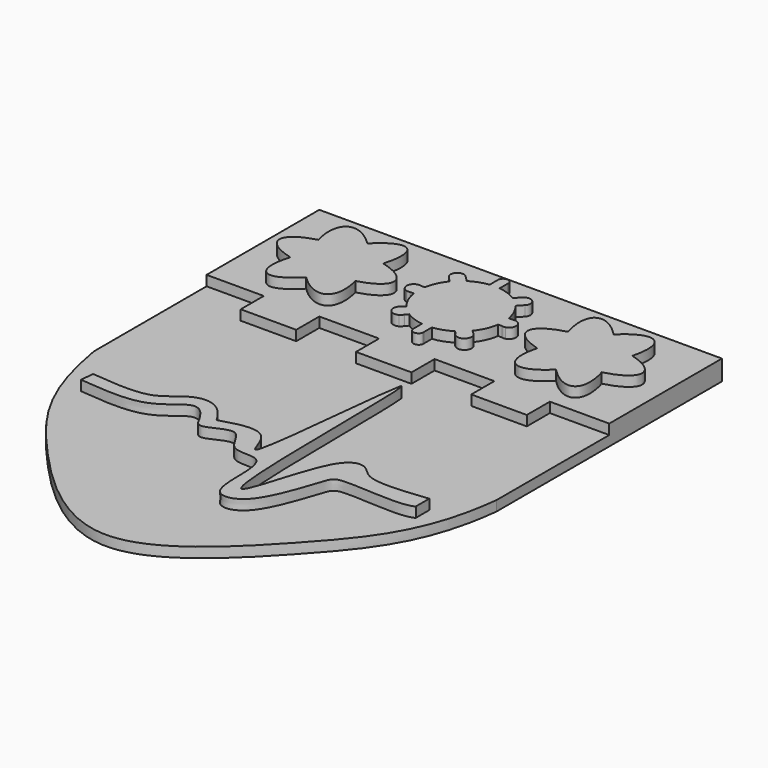
from build123d import *

# Parameters (mm, degrees)
F1_W     = 39.9420261383
F1_H     = 27.9453219846
F2_DEPTH = 1
F4_DEPTH = 1
F6_DEPTH = 1


# Not quite as in the source:
# - the dataset's text gives a spline's control points without its knots; the knots are read off the source's solid


with BuildPart() as f2:
    # F1 (on Top) → F2 (new body)
    with BuildSketch(Plane.XY):
        with Locations((-83.5190042853, -4.0500960313)):
            Rectangle(F1_W, F1_H)
        with BuildLine():
            Line((-63.5479912162, -18.0227570236), (-103.4900173545, -18.0227570236))
            add(Edge.make_bspline(
                [(-103.4900173545, -18.0227570236), (-102.2234410048, -25.4669263959), (-97.486988461, -32.1768391347), (-83.4606816135, -46.0047948801), (-69.8215316304, -32.1663174955), (-64.4036382437, -25.4669263959), (-63.5479912162, -18.0227570236)],
                knots=[0, 0, 0, 0, 0.2558847419, 0.5000748483, 0.7439617176, 1, 1, 1, 1], degree=3))
        make_face()
    extrude(amount=F2_DEPTH)

    # F3 (on face) → F4 (join)
    with BuildSketch(Plane.XY.offset(1)):
        Polygon((-63.5479912162, -4.0500960313), (-63.5479912162, 9.922564961), (-103.4900173545, 9.922564961), (-103.4900173545, -4.0500960313), (-97.8155806661, -4.0500960313), (-97.8155806661, -6.9113592617), (-92.309743166, -6.9113592617), (-92.309743166, -4.0500960313), (-86.3803848624, -4.0500960313), (-86.3803848624, -6.9113592617), (-80.8745473623, -6.9113592617), (-80.8745473623, -4.0500960313), (-74.9451816082, -4.0500960313), (-74.9451816082, -6.9113592617), (-69.4393441081, -6.9113592617), (-69.4393441081, -4.0500960313), align=None)
        with BuildLine():
            add(Edge.make_bspline(
                [(-99.9630689621, -22.528225556), (-97.8050084092, -22.7383123223), (-94.1912663782, -23.0901093914), (-92.2422886498, -20.9561810285), (-90.3592675898, -20.2382765916), (-88.6710398016, -21.005893073), (-88.0005728108, -22.0533678663), (-87.6555964351, -22.5923266262)],
                knots=[0, 0, 0, 0, 0.2982120175, 0.4993656458, 0.66799691, 0.8291739574, 1, 1, 1, 1], degree=3))
            Line((-99.9630689621, -22.528225556), (-100.0935046569, -23.8680916157))
            add(Edge.make_bspline(
                [(-100.0935046569, -23.8680916157), (-99.641213077, -23.9121221112), (-98.7256666906, -24.0013256025), (-97.3584195596, -24.0992161028), (-96.2496019484, -24.1156934281), (-95.3896884341, -24.0638057393), (-94.7581929451, -23.9828672575), (-94.1422492867, -23.8502276061), (-93.5344705995, -23.6422045902), (-93.006004873, -23.3810911586), (-92.5512837964, -23.0968639007), (-92.1638061399, -22.8137321841), (-91.8333347735, -22.5526394177), (-91.5990504655, -22.367477718), (-91.4335751937, -22.2442966641), (-91.3220361628, -22.1663504456), (-91.2159956347, -22.0984600773), (-91.0759198908, -22.0169760478), (-90.9085588347, -21.9349451245), (-90.7257093459, -21.8681143195), (-90.5668189159, -21.8310155496), (-90.4352776818, -21.8190847483), (-90.290771702, -21.8270624276), (-90.0603195544, -21.8881208906), (-89.8056183823, -22.0372246709), (-89.6190164707, -22.1952265623), (-89.420072284, -22.4014685652), (-89.1509209686, -22.7543702908), (-88.9156376248, -23.1208761097), (-88.789421369, -23.3180645593)],
                knots=[0, 0, 0, 0, 0.0625, 0.125, 0.1875, 0.21875, 0.25, 0.28125, 0.3125, 0.34375, 0.375, 0.40625, 0.4375, 0.46875, 0.484375, 0.5, 0.515625, 0.53125, 0.5625, 0.59375, 0.625, 0.65625, 0.6875, 0.75, 0.8125, 0.84375, 0.875, 0.9375, 1, 1, 1, 1], degree=3))
            add(Edge.make_bspline(
                [(-88.789421369, -23.3180645593), (-88.6064399588, -23.7055464069), (-88.1334203276, -24.7072138465), (-84.8867718058, -22.1498784727), (-84.1139103536, -26.1676816962), (-80.4918087102, -24.9787016454), (-80.5104213919, -29.1352666664), (-80.3521996357, -32.500651404), (-76.6927369801, -31.9827435011), (-74.8542261683, -25.2740014974), (-74.103136335, -24.0138444224), (-67.6515141347, -24.9719990423), (-66.5661245584, -24.263119325)],
                knots=[0, 0, 0, 0, 0.0560038879, 0.1447739329, 0.2315937968, 0.3157568277, 0.4138471485, 0.5050737567, 0.5873258169, 0.7241585594, 0.7883299015, 0.9309694647, 0.9309694647, 0.9309694647, 0.9309694647], degree=3))
            Line((-66.5661245584, -24.263119325), (-66.566221416, -22.5923266262))
            add(Edge.make_bspline(
                [(-87.6555964351, -22.5923266262), (-85.892468446, -22.0624948678), (-82.88294857, -21.1581140072), (-81.8661255421, -28.9674864594), (-79.189868147, 7.6035712637), (-80.2972010381, -41.1991140851), (-76.7122142141, -21.5352294093), (-73.6666754342, -21.215900503), (-72.5063764781, -23.2421096322), (-68.8986686121, -22.84746888), (-66.566221416, -22.5923266262)],
                knots=[0, 0, 0, 0, 0.1037610874, 0.1771119606, 0.3711377094, 0.59782823, 0.7400426838, 0.8156894581, 0.880839962, 1, 1, 1, 1], degree=3))
        make_face()
    extrude(amount=F4_DEPTH)

    # F5 (on face) → F6 (join)
    with BuildSketch(Plane.XY.offset(2)):
        with BuildLine():
            Line((-84.1366667768, 7.8781278824), (-84.1366667768, 6.858777233))
            ThreePointArc((-84.1366667768, 6.858777233), (-85.0572011542, 6.6404288094), (-85.9061185607, 6.2228179727))
            Line((-85.9061185607, 6.2228179727), (-86.4581018686, 6.7794057541))
            ThreePointArc((-86.4581018686, 6.7794057541), (-87.3759640381, 6.8133999594), (-87.4099582434, 5.8955377899))
            Line((-87.4099582434, 5.8955377899), (-86.8975441343, 5.3410891578))
            ThreePointArc((-86.8975441343, 5.3410891578), (-87.4719753565, 4.4198086549), (-87.7927983621, 3.3826000967))
            Line((-87.7927983621, 3.3826000967), (-88.1761113279, 3.3826000967))
            Line((-88.1761113279, 3.3826000967), (-88.5431246809, 3.3826000967))
            ThreePointArc((-88.5431246809, 3.3826000967), (-89.0536756709, 2.7132411914), (-88.5431246809, 2.0438822861))
            Line((-88.5431246809, 2.0438822861), (-88.1761113279, 2.0438822861))
            Line((-88.1761113279, 2.0438822861), (-87.8090979749, 2.0438822861))
            ThreePointArc((-87.8090979749, 2.0438822861), (-87.4973115519, 0.9615627135), (-86.9107763195, 0))
            Line((-86.9107763195, 0), (-87.1603672814, -0.2590857621))
            Line((-87.1603672814, -0.2590857621), (-87.4099582434, -0.5181715242))
            ThreePointArc((-87.4099582434, -0.5181715242), (-87.2984320103, -1.3613590557), (-86.4581018686, -1.4926928561))
            Line((-86.4581018686, -1.4926928561), (-86.1458345887, -1.1629684669))
            Line((-86.1458345887, -1.1629684669), (-85.8991036613, -0.9024441994))
            ThreePointArc((-85.8991036613, -0.9024441994), (-85.0532840762, -1.3169808866), (-84.1366667768, -1.5339236488))
            ThreePointArc((-84.1366667768, -1.5339236488), (-83.6444095367, -1.5646709428), (-83.1519216299, -1.5378707908))
            ThreePointArc((-83.1519216299, -1.5378707908), (-82.2176100855, -1.3226639626), (-81.3558285635, -0.9024441994))
            Line((-81.3558285635, -0.9024441994), (-81.109097636, -1.1629684669))
            Line((-81.109097636, -1.1629684669), (-80.7968303561, -1.4926928561))
            ThreePointArc((-80.7968303561, -1.4926928561), (-79.9565002145, -1.3613590557), (-79.8449739814, -0.5181715242))
            Line((-79.8449739814, -0.5181715242), (-80.0945649433, -0.2590857621))
            Line((-80.0945649433, -0.2590857621), (-80.3441559052, 0))
            ThreePointArc((-80.3441559052, 0), (-79.7576206729, 0.9615627135), (-79.4458342499, 2.0438822861))
            Line((-79.4458342499, 2.0438822861), (-79.0788208968, 2.0438822861))
            Line((-79.0788208968, 2.0438822861), (-78.7118075438, 2.0438822861))
            ThreePointArc((-78.7118075438, 2.0438822861), (-78.2012565538, 2.7132411914), (-78.7118075438, 3.3826000967))
            Line((-78.7118075438, 3.3826000967), (-79.0788208968, 3.3826000967))
            Line((-79.0788208968, 3.3826000967), (-79.4621338626, 3.3826000967))
            ThreePointArc((-79.4621338626, 3.3826000967), (-79.7829568683, 4.4198086549), (-80.3573880904, 5.3410891578))
            Line((-80.3573880904, 5.3410891578), (-79.8449739814, 5.8955377899))
            ThreePointArc((-79.8449739814, 5.8955377899), (-79.8789681867, 6.8133999594), (-80.7968303561, 6.7794057541))
            Line((-80.7968303561, 6.7794057541), (-81.348813664, 6.2228179727))
            ThreePointArc((-81.348813664, 6.2228179727), (-82.2136874047, 6.6461275973), (-83.1519216299, 6.862724375))
            Line((-83.1519216299, 6.862724375), (-83.1519216299, 7.8497258035))
            Line((-83.1519216299, 7.8497258035), (-83.1519216299, 7.9462644644))
            ThreePointArc((-83.1519216299, 7.9462644644), (-83.6575465966, 8.3915449283), (-84.1366667768, 7.9178623855))
            Line((-84.1366667768, 7.9178623855), (-84.1366667768, 7.8781278824))
        make_face()
        with BuildLine():
            ThreePointArc((-84.1366667768, 7.9178623855), (-84.1370666386, 7.8979951339), (-84.1366667768, 7.8781278824))
            Line((-84.1366667768, 7.8781278824), (-84.1366667768, 7.9178623855))
        make_face()
        with BuildLine():
            ThreePointArc((-83.1519216299, 7.8497258035), (-83.1495565687, 7.8979951339), (-83.1519216299, 7.9462644644))
            Line((-83.1519216299, 7.9462644644), (-83.1519216299, 7.8497258035))
        make_face()
        with BuildLine():
            Line((-88.5431246809, 3.3826000967), (-88.1761113279, 3.3826000967))
            ThreePointArc((-88.1761113279, 3.3826000967), (-88.3596180044, 3.4072988579), (-88.5431246809, 3.3826000967))
        make_face()
        with BuildLine():
            Line((-88.1761113279, 2.0438822861), (-88.5431246809, 2.0438822861))
            ThreePointArc((-88.5431246809, 2.0438822861), (-88.3596180044, 2.0191835249), (-88.1761113279, 2.0438822861))
        make_face()
        with BuildLine():
            ThreePointArc((-78.7118075438, 3.3826000967), (-78.8953142203, 3.4072988579), (-79.0788208968, 3.3826000967))
            Line((-79.0788208968, 3.3826000967), (-78.7118075438, 3.3826000967))
        make_face()
        with BuildLine():
            Line((-87.4099582434, -0.5181715242), (-87.1603672814, -0.2590857621))
            ThreePointArc((-87.1603672814, -0.2590857621), (-87.3018426282, -0.3725600498), (-87.4099582434, -0.5181715242))
        make_face()
        with BuildLine():
            ThreePointArc((-79.0788208968, 2.0438822861), (-78.8953142203, 2.0191835249), (-78.7118075438, 2.0438822861))
            Line((-78.7118075438, 2.0438822861), (-79.0788208968, 2.0438822861))
        make_face()
        with BuildLine():
            Line((-86.1458345887, -1.1629684669), (-86.4581018686, -1.4926928561))
            ThreePointArc((-86.4581018686, -1.4926928561), (-86.2748984269, -1.3534672648), (-86.1458345887, -1.1629684669))
        make_face()
        with BuildLine():
            ThreePointArc((-83.1519216299, -1.5378707908), (-83.6444095367, -1.5646709428), (-84.1366667768, -1.5339236488))
            Line((-84.1366667768, -1.5339236488), (-84.1366667768, -2.5532742982))
            Line((-84.1366667768, -2.5532742982), (-84.1366667768, -2.5930088013))
            ThreePointArc((-84.1366667768, -2.5930088013), (-83.6575465966, -3.0666913442), (-83.1519216299, -2.6214108802))
            Line((-83.1519216299, -2.6214108802), (-83.1519216299, -2.5248722193))
            Line((-83.1519216299, -2.5248722193), (-83.1519216299, -1.5378707908))
        make_face()
        with BuildLine():
            ThreePointArc((-79.8449739814, -0.5181715242), (-79.9530895966, -0.3725600498), (-80.0945649433, -0.2590857621))
            Line((-80.0945649433, -0.2590857621), (-79.8449739814, -0.5181715242))
        make_face()
        with BuildLine():
            Line((-84.1366667768, -2.5930088013), (-84.1366667768, -2.5532742982))
            ThreePointArc((-84.1366667768, -2.5532742982), (-84.1370666386, -2.5731415498), (-84.1366667768, -2.5930088013))
        make_face()
        with BuildLine():
            ThreePointArc((-83.1519216299, -2.6214108802), (-83.1495565687, -2.5731415498), (-83.1519216299, -2.5248722193))
            Line((-83.1519216299, -2.5248722193), (-83.1519216299, -2.6214108802))
        make_face()
        with BuildLine():
            ThreePointArc((-81.109097636, -1.1629684669), (-80.9800337978, -1.3534672648), (-80.7968303561, -1.4926928561))
            Line((-80.7968303561, -1.4926928561), (-81.109097636, -1.1629684669))
        make_face()
        with BuildLine():
            add(Edge.make_bspline(
                [(-95.8447667684, 6.3409966435), (-101.1057906311, 11.5573827987), (-99.2071204859, 4.4427292948)],
                knots=[2.153396002, 2.153396002, 2.153396002, 4.1180410694, 4.1180410694, 4.1180410694], degree=2, weights=[1, 0.555092188, 1]))
            add(Edge.make_bspline(
                [(-99.2071204859, 4.4427292948), (-105.9961635461, 2.5895118637), (-99.0709977986, 0.8133108115)],
                knots=[5.326754781, 5.326754781, 5.326754781, 7.2686395089, 7.2686395089, 7.2686395089], degree=2, weights=[1, 0.5645219377, 1]))
            add(Edge.make_bspline(
                [(-99.0709977986, 0.8133108115), (-101.245642949, -6.4587366342), (-96.0185316477, -1.0489321332)],
                knots=[2.1459957755, 2.1459957755, 2.1459957755, 4.1205536129, 4.1205536129, 4.1205536129], degree=2, weights=[1, 0.5509627211, 1]))
            add(Edge.make_bspline(
                [(-96.0185316477, -1.0489321332), (-90.7575077851, -6.2653182885), (-92.6561779302, 0.8493352154)],
                knots=[5.2949886556, 5.2949886556, 5.2949886556, 7.259633723, 7.259633723, 7.259633723], degree=2, weights=[1, 0.555092188, 1]))
            add(Edge.make_bspline(
                [(-92.6561779302, 0.8493352154), (-85.8671348701, 2.7025526465), (-92.7923006176, 4.4787536988)],
                knots=[2.1851621274, 2.1851621274, 2.1851621274, 4.1270468554, 4.1270468554, 4.1270468554], degree=2, weights=[1, 0.5645219377, 1]))
            add(Edge.make_bspline(
                [(-92.7923006176, 4.4787536988), (-90.6176554671, 11.7508011445), (-95.8447667684, 6.3409966435)],
                knots=[5.2875884291, 5.2875884291, 5.2875884291, 7.2621462665, 7.2621462665, 7.2621462665], degree=2, weights=[1, 0.5509627211, 1]))
        make_face()
        with BuildLine():
            add(Edge.make_bspline(
                [(-68.0478117389, 4.4427292948), (-66.1491415937, 11.5573827987), (-71.4101654564, 6.3409966435)],
                knots=[2.1651442378, 2.1651442378, 2.1651442378, 4.1297893052, 4.1297893052, 4.1297893052], degree=2, weights=[1, 0.555092188, 1]))
            add(Edge.make_bspline(
                [(-71.4101654564, 6.3409966435), (-76.6372767576, 11.7508011445), (-74.4626316072, 4.4787536988)],
                knots=[5.3042243479, 5.3042243479, 5.3042243479, 7.2787821853, 7.2787821853, 7.2787821853], degree=2, weights=[1, 0.5509627211, 1]))
            add(Edge.make_bspline(
                [(-74.4626316072, 4.4787536988), (-81.3877973547, 2.7025526465), (-74.5987542945, 0.8493352154)],
                knots=[2.1561384518, 2.1561384518, 2.1561384518, 4.0980231798, 4.0980231798, 4.0980231798], degree=2, weights=[1, 0.5645219377, 1]))
            add(Edge.make_bspline(
                [(-74.5987542945, 0.8493352154), (-76.4974244397, -6.2653182885), (-71.236400577, -1.0489321332)],
                knots=[5.3067368914, 5.3067368914, 5.3067368914, 7.2713819588, 7.2713819588, 7.2713819588], degree=2, weights=[1, 0.555092188, 1]))
            add(Edge.make_bspline(
                [(-71.236400577, -1.0489321332), (-66.0092892757, -6.4587366342), (-68.1839344262, 0.8133108115)],
                knots=[2.1626316943, 2.1626316943, 2.1626316943, 4.1371895317, 4.1371895317, 4.1371895317], degree=2, weights=[1, 0.5509627211, 1]))
            add(Edge.make_bspline(
                [(-68.1839344262, 0.8133108115), (-61.2587686787, 2.5895118637), (-68.0478117389, 4.4427292948)],
                knots=[5.2977311054, 5.2977311054, 5.2977311054, 7.2396158334, 7.2396158334, 7.2396158334], degree=2, weights=[1, 0.5645219377, 1]))
        make_face()
    extrude(amount=F6_DEPTH)


solid = f2.part
